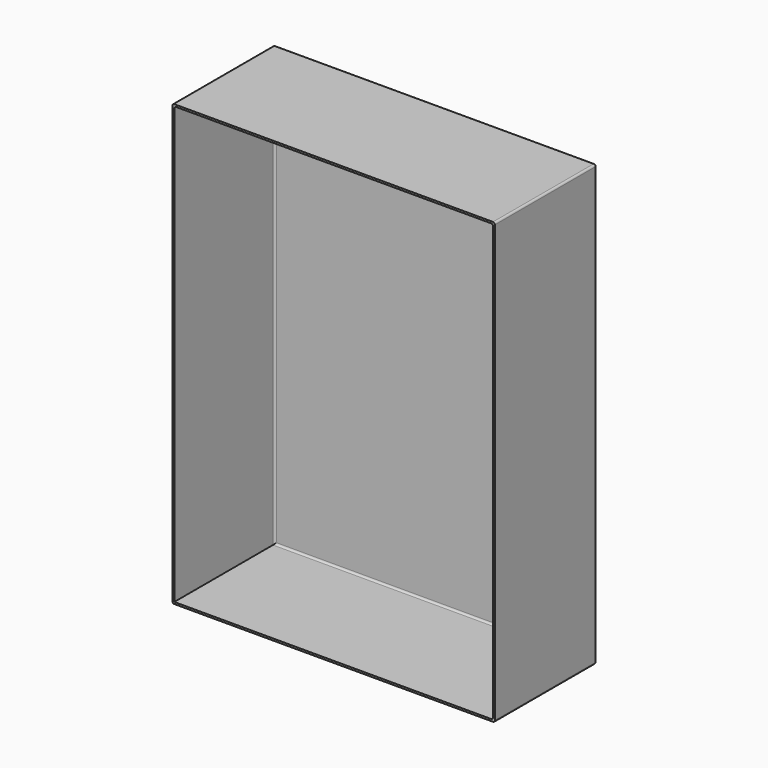
from build123d import *

# Parameters (mm, degrees)
F0_W     = 170
F0_H     = 232
F1_DEPTH = 67
F2_T     = -1
F3_R     = 1


with BuildPart() as f1:
    # F0 (on Front) → F1 (new body)
    with BuildSketch(Plane.XZ):
        Rectangle(F0_W, F0_H)
    extrude(amount=F1_DEPTH)

    # F2
    f2_openings = [f1.faces().sort_by_distance(p)[0] for p in [
        (0, -67, 0),
    ]]
    offset(amount=F2_T, openings=f2_openings)

    # F3
    f3_edges = [f1.edges().sort_by_distance(p)[0] for p in [
        (85, -33.5, -116),
        (85, -33.5, 116),
        (85, 0, 0),
        (0, 0, -116),
        (-85, 0, 0),
        (-85, -33.5, -116),
        (-85, -33.5, 116),
        (0, 0, 116),
        (84, -34, 115),
        (0, -1, -115),
        (84, -1, 0),
        (0, -1, 115),
        (-84, -1, 0),
        (84, -34, -115),
        (-84, -34, 115),
    ]]
    fillet(f3_edges, radius=F3_R)


solid = f1.part
